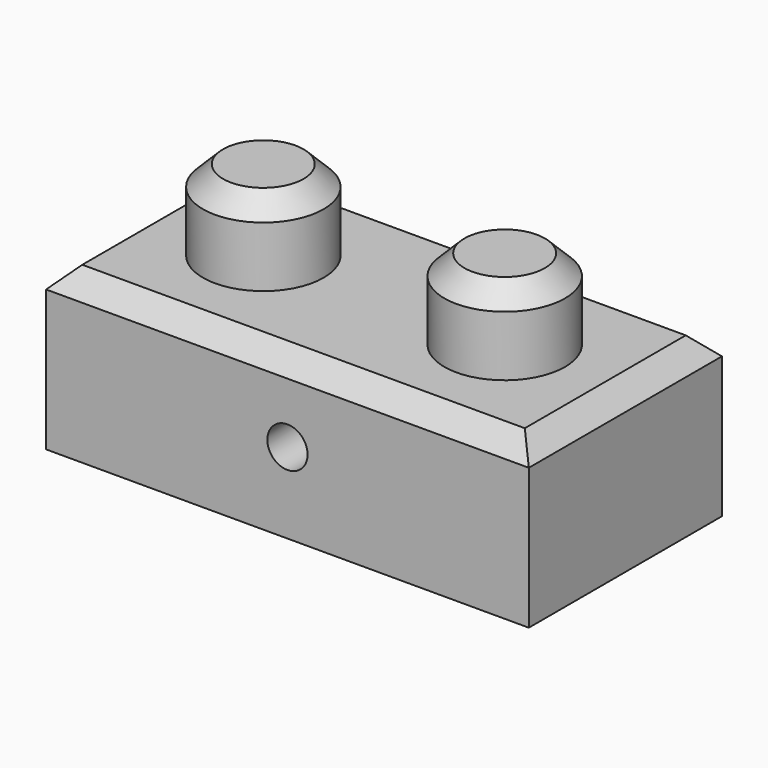
from build123d import *

# Parameters (mm, degrees)
F0_W     = 76.2
F0_H     = 38.1
F1_DEPTH = 25.4
F2_R     = 9.525
F3_DEPTH = 12.7
F4_SIZE2 = 3.175
F4_SIZE  = 3.175
F5_T     = 7.9375
F6_R     = 3.175
F7_DEPTH = 38.1


# Not quite as in the source:
# - a shell that OpenCascade refuses in one call is made with other operations: the cavity is built on its own and cut out


with BuildPart() as f1:
    # F0 (on Top) → F1 (new body)
    with BuildSketch(Plane.XY):
        with Locations((38.1, -19.05)):
            Rectangle(F0_W, F0_H)
    extrude(amount=F1_DEPTH)

    # F2 (on face) → F3 (join)
    with BuildSketch(Plane.XY.offset(25.4)):
        with Locations((57.15, -19.05)):
            Circle(F2_R)
        with Locations((19.05, -19.05)):
            Circle(F2_R)
    extrude(amount=F3_DEPTH)

    # F4
    f4_edges = [f1.edges().sort_by_distance(p)[0] for p in [
        (9.525, -19.05, 38.1),
        (47.625, -19.05, 38.1),
        (76.2, -19.05, 25.4),
        (38.1, -38.1, 25.4),
        (0, -19.05, 25.4),
        (38.1, 0, 25.4),
    ]]
    chamfer(f4_edges, length=F4_SIZE, length2=F4_SIZE2)

    # F5: shell of thickness 7.9375, made by hand


with BuildPart() as f5_core1:
    # F5_t2: copy of F1
    add(f1.part)

    # the walls: a layer under each face that stays
    f5_faces = [f5_core1.faces().sort_by_distance(p)[0] for p in [
        (38.1, 0, 11.1125),
        (76.2, -19.05, 11.1125),
        (38.1, -1.5875, 23.8125),
        (0, -19.05, 11.1125),
        (38.1, -38.1, 11.1125),
        (74.6125, -19.05, 23.8125),
        (38.1, -19.05, 25.4),
        (1.5875, -19.05, 23.8125),
        (38.1, -36.5125, 23.8125),
        (9.525, -19.05, 30.1625),
        (47.625, -19.05, 30.1625),
        (11.1125, -19.05, 36.5125),
        (49.2125, -19.05, 36.5125),
        (19.05, -19.05, 38.1),
        (57.15, -19.05, 38.1),
    ]]
    thicken(f5_faces, amount=-F5_T, mode=Mode.SUBTRACT)

    # F5_s3 → F5_t4 (revolve, cut)
    with BuildSketch(Plane.XZ.offset(19.05)):
        Polygon((28.654375, 25.479375), (28.575, 17.4625), (20.6375, 17.4625), (20.6375, 25.4), align=None)
    revolve(axis=Axis((19.05, -19.05, 25.4), (0, 0, 1)), mode=Mode.SUBTRACT)

    # F5_s5 → F5_t6 (revolve, cut)
    with BuildSketch(Plane.XZ.offset(19.05)):
        Polygon((66.754375, 25.479375), (66.675, 17.4625), (58.7375, 17.4625), (58.7375, 25.4), align=None)
    revolve(axis=Axis((57.15, -19.05, 25.4), (0, 0, 1)), mode=Mode.SUBTRACT)


with BuildPart() as f1_1:
    add(f1.part)

    # what is left inside the walls is the cavity
    f5_cavity = [f5_core1.part.solids().sort_by_distance(p)[0] for p in [
        (38.1, -22.754167, 0.079375),
    ]]
    add(f5_cavity, mode=Mode.SUBTRACT)

    # F6 (on face) → F7 (cut)
    with BuildSketch(Plane.XZ.offset(38.1)):
        with Locations((38.1, 12.7)):
            Circle(F6_R)
    extrude(amount=-F7_DEPTH, mode=Mode.SUBTRACT)


solid = f1_1.part
